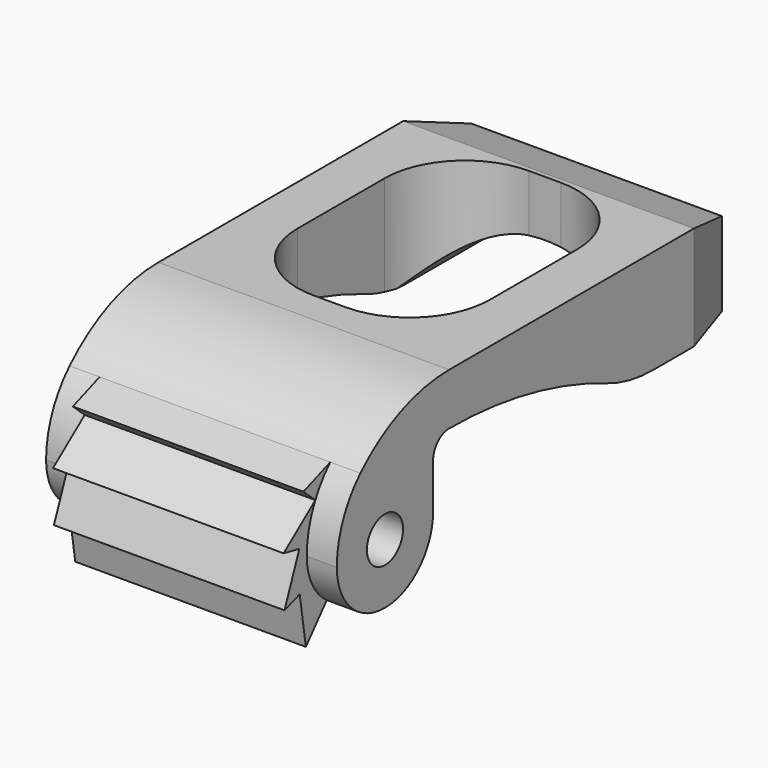
from build123d import *

# Parameters (mm, degrees)
F1_R      = 1.7859375
F2_DEPTH  = 3.96875
F3_DEPTH  = 9.128125
F4_START  = 9.128125
F0_R      = 1.7859375
F4_DEPTH  = 2.38125
F7_DEPTH  = 11.509375
F6_W      = 15.24
F6_H      = 21.336
F8_DEPTH  = 9.2536280605
F9_R      = 6.35
F11_DEPTH = 10.4116969269
F12_SIZE2 = 4.7625
F12_SIZE  = 1.5875


# Not quite as in the source:
# - a feature names something its author has since deleted; it is built from what else it names


with BuildPart() as f2:
    # F1 (on Right) → F2 (new body, symmetric)
    with BuildSketch(Plane.YZ):
        with BuildLine():
            Line((-3.4820551441, -0.7959792641), (-2.7800674169, -3.8668632517))
            ThreePointArc((-2.7800674169, -3.8668632517), (2.1727097341, -4.2380111682), (4.7625, 0))
            Line((4.7625, 0), (4.7625, 3.571875))
            Line((4.7625, 3.571875), (0, 3.571875))
            ThreePointArc((0, 3.571875), (-2.7929759621, 2.2265615399), (-3.4820551441, -0.7959792641))
        make_face()
        Circle(F1_R, mode=Mode.SUBTRACT)
    extrude(amount=F2_DEPTH, both=True)

    # F1 (on Right) → F3 (join, symmetric)
    with BuildSketch(Plane.YZ):
        with BuildLine():
            Line((-6.9643447844, -2.8750519268), (-5.4621269675, -2.3617314805))
            Line((-5.4621269675, -2.3617314805), (-4.8504655451, -6.2830637627))
            Line((-4.8504655451, -6.2830637627), (-3.8175156986, -5.077588394))
            Line((-3.8175156986, -5.077588394), (-2.7800674169, -3.8668632517))
            Line((-2.7800674169, -3.8668632517), (-3.4820551441, -0.7959792641))
            ThreePointArc((-3.4820551441, -0.7959792641), (-2.7929759621, 2.2265615399), (0, 3.571875))
            Line((0, 3.571875), (4.7625, 3.571875))
            ThreePointArc((4.7625, 3.571875), (5.2274679849, 4.6944070151), (6.35, 5.159375))
            Line((6.35, 5.159375), (6.35, 9.2526280605))
            ThreePointArc((6.35, 9.2526280605), (1.5941526376, 8.3066312028), (-2.4376600757, 5.6126600757))
            Line((-2.4376600757, 5.6126600757), (-5.0921494321, 4.6325641503))
            Line((-5.0921494321, 4.6325641503), (-3.9164474257, 3.5658490795))
            Line((-3.9164474257, 3.5658490795), (-7.0531168828, 1.134330772))
            Line((-7.0531168828, 1.134330772), (-5.4984652486, 0.8130605645))
            Line((-5.4984652486, 0.8130605645), (-6.9643447844, -2.8750519268))
        make_face()
    extrude(amount=F3_DEPTH, both=True)

    # F0 (on Right) → F4 (join)
    with BuildSketch(Plane.YZ.offset(F4_START)):
        with BuildLine():
            ThreePointArc((-2.4376600757, 5.6126600757), (-4.1582937893, 3.0375497444), (-4.7625, 0))
            ThreePointArc((-4.7625, 0), (0, -4.7625), (4.7625, 0))
            Line((4.7625, 0), (4.7625, 3.571875))
            ThreePointArc((4.7625, 3.571875), (5.2274679849, 4.6944070151), (6.35, 5.159375))
            Line((6.35, 5.159375), (6.35, 9.2526280605))
            ThreePointArc((6.35, 9.2526280605), (1.5941526376, 8.3066312028), (-2.4376600757, 5.6126600757))
        make_face()
        Circle(F0_R, mode=Mode.SUBTRACT)
    extrude(amount=F4_DEPTH)


with BuildPart() as f5_1:
    # F5: instance of F2
    add(f2.part.mirror(Plane.YZ))


with BuildPart() as f2_1:
    add(f2.part)

    add(f5_1.part)  # F7 merges F5_1
    # F0 (on Right) → F7 (join, symmetric)
    with BuildSketch(Plane.YZ):
        with BuildLine():
            Line((35.3293530643, 9.2526280605), (6.35, 9.2526280605))
            Line((6.35, 9.2526280605), (6.35, 5.159375))
            ThreePointArc((6.35, 5.159375), (14.3027763595, 4.3544032669), (21.9329443326, 1.9721421521))
            ThreePointArc((21.9329443326, 1.9721421521), (24.1912770347, 1.2670543743), (26.5450934892, 1.0288035264))
            Line((26.5450934892, 1.0288035264), (35.3293530643, 1.0288035264))
            Line((35.3293530643, 1.0288035264), (35.3293530643, 9.2526280605))
        make_face()
    extrude(amount=F7_DEPTH, both=True)

    # F6 (on Top) → F8 (cut, through all)
    with BuildSketch(Plane.XY):
        with Locations((0, 19.558)):
            Rectangle(F6_W, F6_H)
    extrude(amount=F8_DEPTH, mode=Mode.SUBTRACT)

    # F9
    f9_edges = [f2_1.edges().sort_by_distance(p)[0] for p in [
        (-7.62, 30.226, 5.140716),
        (7.62, 30.226, 5.140716),
        (7.62, 8.89, 7.16532),
        (-7.62, 8.89, 7.16532),
    ]]
    fillet(f9_edges, radius=F9_R)

    # F10 (on face) → F11 (cut, through all)
    with BuildSketch(Plane(origin=(0, 35.3293530643, 0), x_dir=(-1, 0, 0), z_dir=(0, 1, 0))):
        with BuildLine():
            Line((-7.62, 1.0288035264), (7.62, 1.0288035264))
            ThreePointArc((7.62, 1.0288035264), (0, 4.8388035264), (-7.62, 1.0288035264))
        make_face()
    extrude(amount=-F11_DEPTH, mode=Mode.SUBTRACT)

    # F12
    f12_edges = [f2_1.edges().sort_by_distance(p)[0] for p in [
        (11.509375, 35.329353, 5.140716),
        (-11.509375, 35.329353, 5.140716),
        (0, 35.329353, 9.252628),
    ]]
    f12_side = f2_1.faces().sort_by_distance((0, 35.329353, 5.838802))[0]
    chamfer(f12_edges, length=F12_SIZE, length2=F12_SIZE2, reference=f12_side)


solid = f2_1.part
